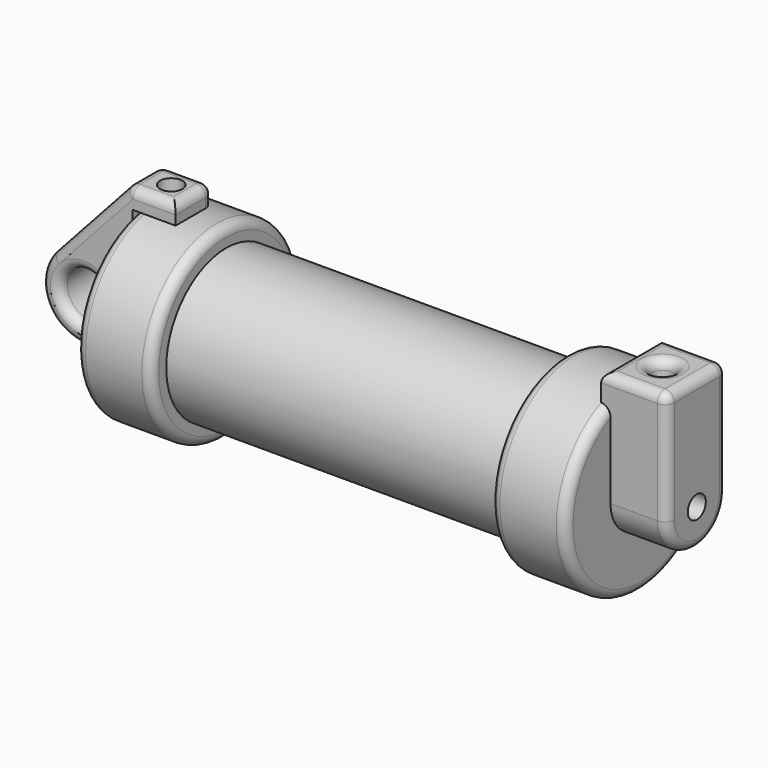
from build123d import *

# Parameters (mm, degrees)
F0_W          = 5.842
F0_H          = 12.7
F0_R          = 3.175
F2_DEPTH      = 3.175
F3_R          = 1.524
F4_DEPTH      = 7.62
F4_DEPTH_BACK = 1.27
F5_R          = 1.524
F6_DEPTH      = 10.414
F7_R          = 1.524
F8_DEPTH      = 17.78
F9_R          = 1.26999
F9_2_R        = 1.26999
F9_3_R        = 1.26999


# Not quite as in the source:
# - a fillet or chamfer is up to 0.001 mm smaller than in the source, because OpenCascade refuses the exact size


with BuildPart() as f1:
    # F0 (on Front) → F1 (revolve)
    with BuildSketch(Plane.XZ):
        Polygon((5.842, 12.7), (5.842, 0), (66.294, 0), (66.294, 12.7), (56.134, 12.7), (56.134, 10.16), (10.16, 10.16), (10.16, 12.7), align=None)
        with Locations((2.921, 6.35)):
            Rectangle(F0_W, F0_H)
    revolve(axis=Axis((33.147, 0, 0), (-1, 0, 0)))

    # F9 (radius 1.27 in the source; OpenCascade refuses exactly that, so slightly less here)
    f9_edges = [f1.edges().sort_by_distance(p)[0] for p in [
        (10.16, 0, -12.7),
        (0, 0, -12.7),
        (66.294, 0, -12.7),
        (56.134, 0, -12.7),
    ]]
    fillet(f9_edges, radius=F9_R)


with BuildPart() as f2:
    # F0 (on Front) → F2 (new body, symmetric)
    with BuildSketch(Plane.XZ):
        with BuildLine():
            Line((-0.9398, 0), (0, 0))
            Line((0, 0), (0, 12.7))
            Line((0, 12.7), (5.842, 12.7))
            Line((5.842, 12.7), (5.842, 15.24))
            Line((5.842, 15.24), (-0.508, 15.24))
            Line((-0.508, 15.24), (-10.8806298187, 3.8475430269))
            ThreePointArc((-10.8806298187, 3.8475430269), (-4.5919612295, 5.3297205562), (-0.9398, 0))
        make_face()
        with BuildLine():
            Line((5.842, 0), (0, 0))
            Line((0, 0), (-0.9398, 0))
            ThreePointArc((-0.9398, 0), (-3.1957909266, -4.5493385486), (-8.1826630726, -5.5069827884))
            Line((-8.1826630726, -5.5069827884), (5.842, -9.398))
            Line((5.842, -9.398), (5.842, 0))
        make_face()
        with BuildLine():
            ThreePointArc((-8.1826630726, -5.5069827884), (-3.1957909266, -4.5493385486), (-0.9398, 0))
            ThreePointArc((-0.9398, 0), (-4.5919612295, 5.3297205562), (-10.8806298187, 3.8475430269))
            ThreePointArc((-10.8806298187, 3.8475430269), (-12.1459778134, -1.5837270034), (-8.1826630726, -5.5069827884))
        make_face()
        with Locations((-6.6548, 0)):
            Circle(F0_R, mode=Mode.SUBTRACT)
    extrude(amount=F2_DEPTH, both=True)

    # F7 (on face) → F8 (cut)
    with BuildSketch(Plane.XY.offset(15.24)):
        with Locations((2.6870968286, 0.0285728838)):
            Circle(F7_R)
    extrude(amount=-F8_DEPTH, mode=Mode.SUBTRACT)

    # F9#2 (radius 1.27 in the source; OpenCascade refuses exactly that, so slightly less here)
    f9_2_edges = [f2.edges().sort_by_distance(p)[0] for p in [
        (2.667, -3.175, 15.24),
        (5.842, 3.175, 13.97),
        (-0.508, 0, 15.24),
        (2.667, 3.175, 15.24),
        (-5.694315, 3.175, 9.543772),
        (-10.88063, 0, 3.847543),
        (-5.694315, -3.175, 9.543772),
        (-9.8298, -3.175, 0),
        (5.842, 0, 15.24),
        (-1.170332, 3.175, -7.452491),
        (-1.170332, -3.175, -7.452491),
        (-12.145978, 3.175, -1.583727),
        (-12.145978, -3.175, -1.583727),
    ]]
    fillet(f9_2_edges, radius=F9_2_R)


with BuildPart() as f4:
    # F3 (on face) → F4 (new body, two sides)
    with BuildSketch(Plane.YZ.offset(66.294)) as f4_sk:
        with BuildLine():
            ThreePointArc((-5.08, 0), (0, -5.08), (5.08, 0))
            ThreePointArc((5.08, 0), (0, 5.08), (-5.08, 0))
        make_face()
        Circle(F3_R, mode=Mode.SUBTRACT)
        with BuildLine():
            ThreePointArc((-5.08, 0), (0, 5.08), (5.08, 0))
            Line((5.08, 0), (5.08, 15.24))
            Line((5.08, 15.24), (-5.08, 15.24))
            Line((-5.08, 15.24), (-5.08, 0))
        make_face()
    extrude(amount=F4_DEPTH)
    extrude(f4_sk.sketch, amount=-F4_DEPTH_BACK)

    # F5 (on face) → F6 (cut)
    with BuildSketch(Plane.XY.offset(15.24)):
        with Locations((69.2305639386, 0.0387020955)):
            Circle(F5_R)
    extrude(amount=-F6_DEPTH, mode=Mode.SUBTRACT)

    # F9#3 (radius 1.27 in the source; OpenCascade refuses exactly that, so slightly less here)
    f9_3_edges = [f4.edges().sort_by_distance(p)[0] for p in [
        (73.914, 5.08, 7.62),
        (73.914, 0, 15.24),
        (69.469, 5.08, 15.24),
        (69.469, -5.08, 15.24),
        (65.024, 0, 15.24),
        (67.706564, 0.038702, 15.24),
        (73.914, 0, -5.08),
        (73.914, -5.08, 7.62),
    ]]
    fillet(f9_3_edges, radius=F9_3_R)


solid = Compound([f1.part, f2.part, f4.part])
